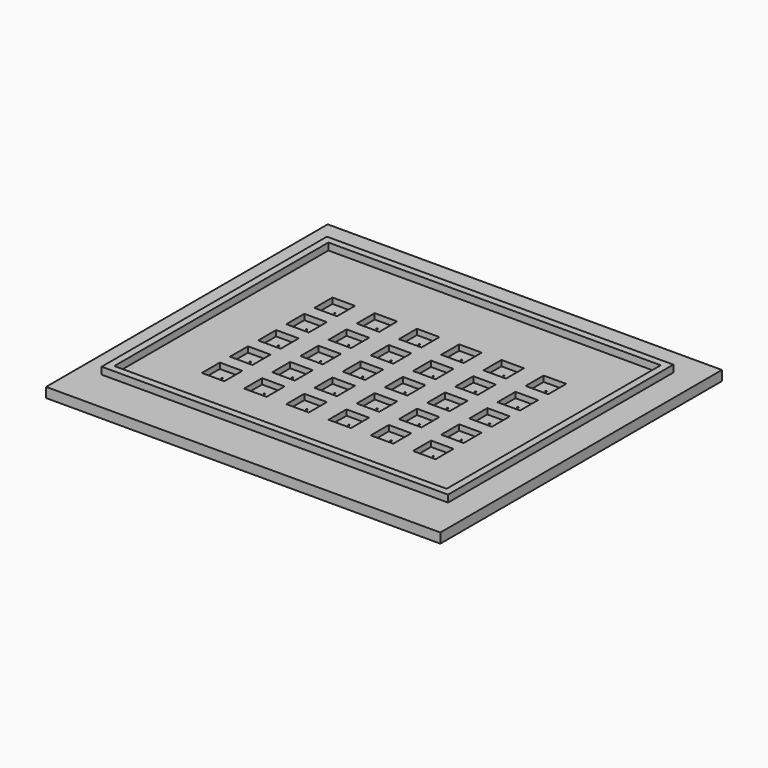
from build123d import *

# Parameters (mm, degrees)
F0_W      = 28
F0_H      = 25
F1_DEPTH  = 0.7
F3_W      = 1.6
F3_H      = 1.6
F4_DEPTH  = 0.4
F6_D      = 0.1
F8_D      = 0.1
F10_D     = 0.1
F12_D     = 0.1
F14_D     = 0.1
F16_D     = 0.1
F18_D     = 0.1
F20_D     = 0.1
F22_D     = 0.1
F24_D     = 0.1
F26_D     = 0.1
F28_D     = 0.1
F30_D     = 0.1
F32_D     = 0.1
F34_D     = 0.1
F36_D     = 0.1
F38_D     = 0.1
F40_D     = 0.1
F42_D     = 0.1
F44_D     = 0.1
F46_D     = 0.1
F48_D     = 0.1
F50_D     = 0.1
F52_D     = 0.1
F54_D     = 0.1
F56_D     = 0.1
F58_D     = 0.1
F60_D     = 0.1
F62_D     = 0.1
F64_D     = 0.1
F2_W      = 24.6
F2_H      = 20
F2_W_2    = 23.599999553
F2_H_2    = 18.999999553
F65_DEPTH = 0.5


# Not quite as in the source:
# - a feature names something its author has since deleted; it is built from what else it names


with BuildPart() as f1:
    # F0 (on Top) → F1 (new body)
    with BuildSketch(Plane.XY):
        Rectangle(F0_W, F0_H)
    extrude(amount=-F1_DEPTH)

    # F3 (on face) → F4 (cut)
    with BuildSketch(Plane.XY):
        with Locations((-7.5, 5)):
            Rectangle(F3_W, F3_H)
        with Locations((-4.5, 5)):
            Rectangle(F3_W, F3_H)
        with Locations((-1.5, 5)):
            Rectangle(F3_W, F3_H)
        with Locations((1.5, 5)):
            Rectangle(F3_W, F3_H)
        with Locations((4.5, 5)):
            Rectangle(F3_W, F3_H)
        with Locations((7.5, 5)):
            Rectangle(F3_W, F3_H)
        with Locations((-7.5, 2.5)):
            Rectangle(F3_W, F3_H)
        with Locations((-4.5, 2.5)):
            Rectangle(F3_W, F3_H)
        with Locations((-1.5, 2.5)):
            Rectangle(F3_W, F3_H)
        with Locations((1.5, 2.5)):
            Rectangle(F3_W, F3_H)
        with Locations((4.5, 2.5)):
            Rectangle(F3_W, F3_H)
        with Locations((7.5, 2.5)):
            Rectangle(F3_W, F3_H)
        with Locations((-7.5, 0)):
            Rectangle(F3_W, F3_H)
        with Locations((-4.5, 0)):
            Rectangle(F3_W, F3_H)
        with Locations((-1.5, 0)):
            Rectangle(F3_W, F3_H)
        with Locations((1.5, 0)):
            Rectangle(F3_W, F3_H)
        with Locations((4.5, 0)):
            Rectangle(F3_W, F3_H)
        with Locations((7.5, 0)):
            Rectangle(F3_W, F3_H)
        with Locations((-7.5, -2.5)):
            Rectangle(F3_W, F3_H)
        with Locations((-4.5, -2.5)):
            Rectangle(F3_W, F3_H)
        with Locations((-1.5, -2.5)):
            Rectangle(F3_W, F3_H)
        with Locations((1.5, -2.5)):
            Rectangle(F3_W, F3_H)
        with Locations((4.5, -2.5)):
            Rectangle(F3_W, F3_H)
        with Locations((7.5, -2.5)):
            Rectangle(F3_W, F3_H)
        with Locations((-7.5, -5)):
            Rectangle(F3_W, F3_H)
        with Locations((-4.5, -5)):
            Rectangle(F3_W, F3_H)
        with Locations((-1.5, -5)):
            Rectangle(F3_W, F3_H)
        with Locations((1.5, -5)):
            Rectangle(F3_W, F3_H)
        with Locations((4.5, -5)):
            Rectangle(F3_W, F3_H)
        with Locations((7.5, -5)):
            Rectangle(F3_W, F3_H)
    extrude(amount=-F4_DEPTH, mode=Mode.SUBTRACT)

    # F6 (through all)
    with Locations(Plane.XY.offset(-0.4)):
        with Locations((-7.5, 5)):
            Hole(F6_D / 2)

    # F8 (through all)
    with Locations(Plane.XY.offset(-0.4)):
        with Locations((-4.5, 5)):
            Hole(F8_D / 2)

    # F10 (through all)
    with Locations(Plane.XY.offset(-0.4)):
        with Locations((-1.5, 5)):
            Hole(F10_D / 2)

    # F12 (through all)
    with Locations(Plane.XY.offset(-0.4)):
        with Locations((1.5, 5)):
            Hole(F12_D / 2)

    # F14 (through all)
    with Locations(Plane.XY.offset(-0.4)):
        with Locations((4.5, 5)):
            Hole(F14_D / 2)

    # F16 (through all)
    with Locations(Plane.XY.offset(-0.4)):
        with Locations((7.5, 5)):
            Hole(F16_D / 2)

    # F18 (through all)
    with Locations(Plane.XY.offset(-0.4)):
        with Locations((7.5, 2.5)):
            Hole(F18_D / 2)

    # F20 (through all)
    with Locations(Plane.XY.offset(-0.4)):
        with Locations((4.5, 2.5)):
            Hole(F20_D / 2)

    # F22 (through all)
    with Locations(Plane.XY.offset(-0.4)):
        with Locations((1.5, 2.5)):
            Hole(F22_D / 2)

    # F24 (through all)
    with Locations(Plane.XY.offset(-0.4)):
        with Locations((-1.5, 2.5)):
            Hole(F24_D / 2)

    # F26 (through all)
    with Locations(Plane.XY.offset(-0.4)):
        with Locations((-4.5, 2.5)):
            Hole(F26_D / 2)

    # F28 (through all)
    with Locations(Plane.XY.offset(-0.4)):
        with Locations((-7.5, 2.5)):
            Hole(F28_D / 2)

    # F30 (through all)
    with Locations(Plane.XY.offset(-0.4)):
        with Locations((-7.5, 0)):
            Hole(F30_D / 2)

    # F32 (through all)
    with Locations(Plane.XY.offset(-0.4)):
        with Locations((-4.5, 0)):
            Hole(F32_D / 2)

    # F34 (through all)
    with Locations(Plane.XY.offset(-0.4)):
        with Locations((-1.5, 0)):
            Hole(F34_D / 2)

    # F36 (through all)
    with Locations(Plane.XY.offset(-0.4)):
        with Locations((1.5, 0)):
            Hole(F36_D / 2)

    # F38 (through all)
    with Locations(Plane.XY.offset(-0.4)):
        with Locations((4.5, 0)):
            Hole(F38_D / 2)

    # F40 (through all)
    with Locations(Plane.XY.offset(-0.4)):
        with Locations((7.5, 0)):
            Hole(F40_D / 2)

    # F42 (through all)
    with Locations(Plane.XY.offset(-0.4)):
        with Locations((-7.5, -2.5)):
            Hole(F42_D / 2)

    # F44 (through all)
    with Locations(Plane.XY.offset(-0.4)):
        with Locations((-4.5, -2.5)):
            Hole(F44_D / 2)

    # F46 (through all)
    with Locations(Plane.XY.offset(-0.4)):
        with Locations((-1.5, -2.5)):
            Hole(F46_D / 2)

    # F48 (through all)
    with Locations(Plane.XY.offset(-0.4)):
        with Locations((1.5, -2.5)):
            Hole(F48_D / 2)

    # F50 (through all)
    with Locations(Plane.XY.offset(-0.4)):
        with Locations((4.5, -2.5)):
            Hole(F50_D / 2)

    # F52 (through all)
    with Locations(Plane.XY.offset(-0.4)):
        with Locations((7.5, -2.5)):
            Hole(F52_D / 2)

    # F54 (through all)
    with Locations(Plane.XY.offset(-0.4)):
        with Locations((7.5, -5)):
            Hole(F54_D / 2)

    # F56 (through all)
    with Locations(Plane.XY.offset(-0.4)):
        with Locations((4.5, -5)):
            Hole(F56_D / 2)

    # F58 (through all)
    with Locations(Plane.XY.offset(-0.4)):
        with Locations((1.5, -5)):
            Hole(F58_D / 2)

    # F60 (through all)
    with Locations(Plane.XY.offset(-0.4)):
        with Locations((-1.5, -5)):
            Hole(F60_D / 2)

    # F62 (through all)
    with Locations(Plane.XY.offset(-0.4)):
        with Locations((-4.5, -5)):
            Hole(F62_D / 2)

    # F64 (through all)
    with Locations(Plane.XY.offset(-0.4)):
        with Locations((-7.5, -5)):
            Hole(F64_D / 2)

    # F2 (on face) → F65 (join)
    with BuildSketch(Plane.XY):
        with Locations((-0.2066325396, 0.5688778237)):
            Rectangle(F2_W, F2_H)
        with Locations((-0.2066325396, 0.5688778237)):
            Rectangle(F2_W_2, F2_H_2, mode=Mode.SUBTRACT)
    extrude(amount=F65_DEPTH)


solid = f1.part
